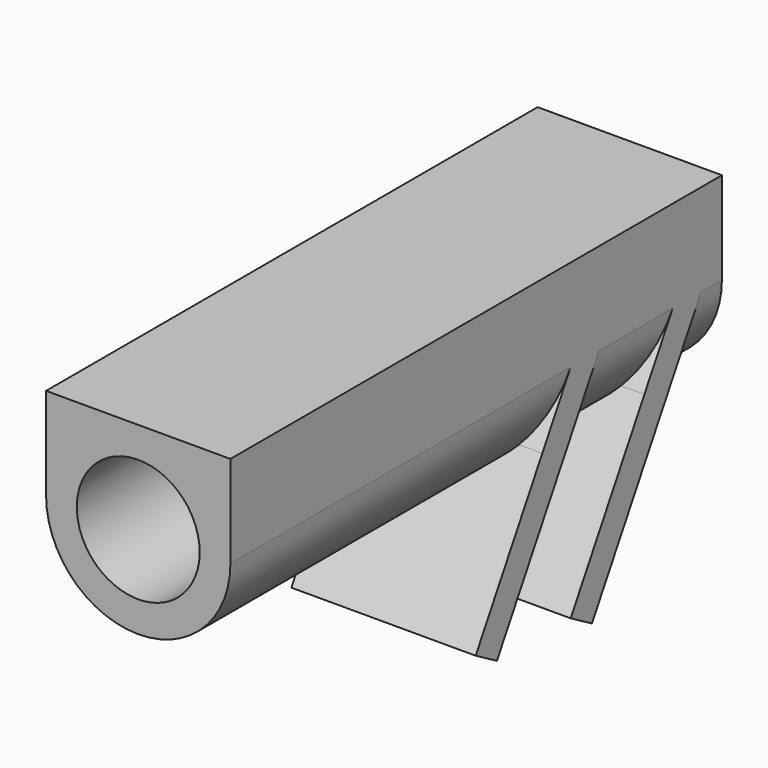
from build123d import *

# Parameters (mm, degrees)
F0_R          = 2
F1_DEPTH      = 20
F3_DEPTH      = 3
F3_DEPTH_BACK = 3
F6_DEPTH      = 1
F9_DEPTH      = 1
F10_DEPTH     = 20


with BuildPart() as f1:
    # F0 (on Front) → F1 (new body)
    with BuildSketch(Plane.XZ):
        with BuildLine():
            ThreePointArc((-3, 0), (0, -3), (3, 0))
            ThreePointArc((3, 0), (2.1213203436, 2.1213203436), (0, 3))
            ThreePointArc((0, 3), (-2.1213203436, 2.1213203436), (-3, 0))
        make_face()
        Circle(F0_R, mode=Mode.SUBTRACT)
    extrude(amount=F1_DEPTH)

    # F2 (on Right) → F3 (join, two sides)
    with BuildSketch(Plane.YZ) as f3_sk:
        Polygon((-5.2886751346, -7.6961524227), (-2, -2), (-3.1547005384, -2), (-6.1547005384, -7.1961524227), align=None)
        Polygon((-9.1547005384, -7.1961524227), (-6.1547005384, -2), (-7.3094010768, -2), (-10.0207259422, -6.6961524227), align=None)
    extrude(amount=F3_DEPTH)
    extrude(f3_sk.sketch, amount=-F3_DEPTH_BACK)

    # F5 (on offset) → F6 (join)
    with BuildSketch(Plane(origin=(0, -0.6339745962, 0.3660254038), x_dir=(-1, 0, 0), z_dir=(0, 0.8660254038, -0.5))):
        Polygon((3, -4), (3, 0), (1.5, -4), align=None)
        Polygon((-1.5, -4), (-3, 0), (-3, -4), align=None)
    extrude(amount=-F6_DEPTH)

    # F8 (on offset) → F9 (join)
    with BuildSketch(Plane(origin=(0, -3.75, 2.1650635095), x_dir=(-1, 0, 0), z_dir=(0, 0.8660254038, -0.5))):
        Polygon((3, -6), (3, -2.5), (1.5, -6), align=None)
        Polygon((-3, -6), (-1.5, -6), (-3, -2.5), align=None)
    extrude(amount=-F9_DEPTH)

    # F0 (on Front) → F10 (join)
    with BuildSketch(Plane.XZ):
        with BuildLine():
            ThreePointArc((-3, 0), (0, -3), (3, 0))
            ThreePointArc((3, 0), (2.1213203436, 2.1213203436), (0, 3))
            ThreePointArc((0, 3), (-2.1213203436, 2.1213203436), (-3, 0))
        make_face()
        Circle(F0_R, mode=Mode.SUBTRACT)
        with BuildLine():
            ThreePointArc((0, 3), (2.1213203436, 2.1213203436), (3, 0))
            Line((3, 0), (3, 3))
            Line((3, 3), (0, 3))
        make_face()
        with BuildLine():
            ThreePointArc((-3, 0), (-2.1213203436, 2.1213203436), (0, 3))
            Line((0, 3), (-3, 3))
            Line((-3, 3), (-3, 0))
        make_face()
    extrude(amount=F10_DEPTH)


solid = f1.part
